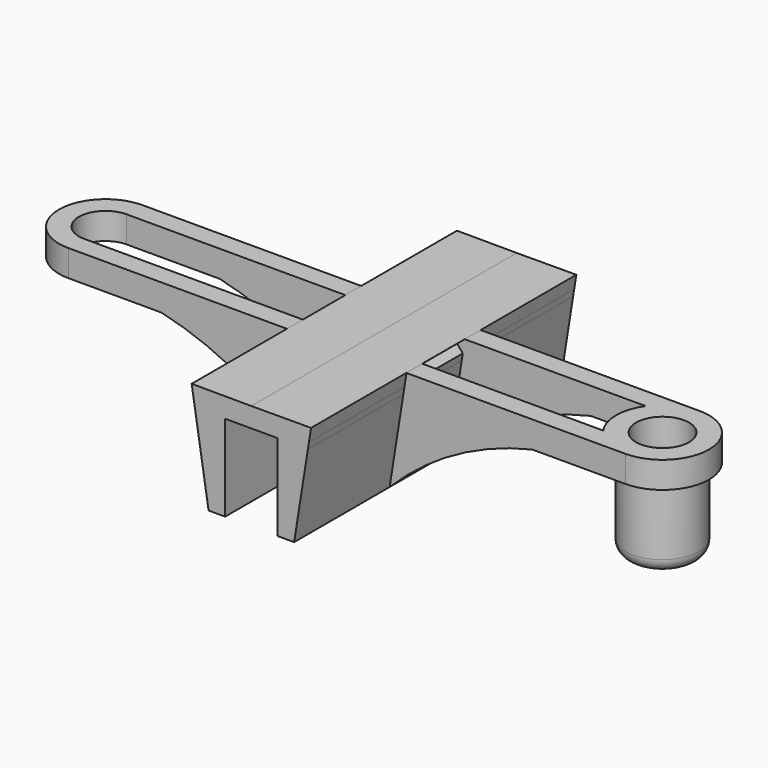
from build123d import *

# Parameters (mm, degrees)
F2_DEPTH  = 25
F3_DEPTH  = 4
F5_R      = 2
F6_DEPTH  = 18
F10_DEPTH = 3
F13_DEPTH = 3


# Not quite as in the source:
# - a feature names something its author has since deleted; it is built from what else it names


with BuildPart() as f2:
    # F0 (on Front) → F2 (new body, symmetric)
    with BuildSketch(Plane.XZ):
        Polygon((-3.95, -2.9709123753), (0, -2.9709123753), (0, 0), (-9, 0.0290876247), (-7.8289458158, -0.965005679), (-8.6815025112, -1.9693279914), (-8.521875, -2.9709123753), align=None)
        Polygon((3.95, -2.9709123753), (8.521875, -2.9709123753), (8.6815025112, -1.9693279914), (7.8289458158, -0.965005679), (9, 0.0290876247), (0, 0), (0, -2.9709123753), align=None)
        Polygon((-3.95, -15.9709123753), (-3.95, -2.9709123753), (-8.521875, -2.9709123753), (-6.45, -15.9709123753), align=None)
        Polygon((3.95, -15.9709123753), (6.45, -15.9709123753), (8.521875, -2.9709123753), (3.95, -2.9709123753), align=None)
    extrude(amount=F2_DEPTH, both=True)



with BuildPart() as f3:
    # F1 (on Top) → F3 (new body)
    with BuildSketch(Plane.XY):
        with BuildLine():
            ThreePointArc((42, -7), (49, 0), (42, 7))
            ThreePointArc((42, 7), (38.7596296508, 6.204836823), (36.2554373535, 4))
            Line((36.2554373535, 4), (42, 4))
            ThreePointArc((42, 4), (46, 0), (42, -4))
            Line((42, -4), (36.2554373535, -4))
            ThreePointArc((36.2554373535, -4), (38.7596296508, -6.204836823), (42, -7))
        make_face()
        with BuildLine():
            Line((7.5, -7), (9, -7))
            Line((9, -7), (42, -7))
            ThreePointArc((42, -7), (38.7596296508, -6.204836823), (36.2554373535, -4))
            Line((36.2554373535, -4), (9, -4))
            Line((9, -4), (7.5, -4))
            Line((7.5, -4), (7.5, -7))
        make_face()
        with BuildLine():
            Line((42, 7), (9, 7))
            Line((9, 7), (7.5, 7))
            Line((7.5, 7), (7.5, 4))
            Line((7.5, 4), (9, 4))
            Line((9, 4), (36.2554373535, 4))
            ThreePointArc((36.2554373535, 4), (38.7596296508, 6.204836823), (42, 7))
        make_face()
        with BuildLine():
            Line((42, 4), (36.2554373535, 4))
            ThreePointArc((36.2554373535, 4), (35, 0), (36.2554373535, -4))
            Line((36.2554373535, -4), (42, -4))
            ThreePointArc((42, -4), (38, 0), (42, 4))
        make_face()
    extrude(amount=-F3_DEPTH)


with BuildPart() as f3b:
    # F1 (on Top) → F3, piece 2 (new body)
    with BuildSketch(Plane.XY):
        with BuildLine():
            Line((-7.5, 7), (-9, 7))
            Line((-9, 7), (-42, 7))
            ThreePointArc((-42, 7), (-49, 0), (-42, -7))
            Line((-42, -7), (-9, -7))
            Line((-9, -7), (-7.5, -7))
            Line((-7.5, -7), (-7.5, -4))
            Line((-7.5, -4), (-9, -4))
            Line((-9, -4), (-42, -4))
            ThreePointArc((-42, -4), (-46, 0), (-42, 4))
            Line((-42, 4), (-9, 4))
            Line((-9, 4), (-7.5, 4))
            Line((-7.5, 4), (-7.5, 7))
        make_face()
    extrude(amount=-F3_DEPTH)


with BuildPart() as f2_1:
    add(f2.part)

    add(f3.part)  # F4 merges F3

    add(f3b.part)  # F4 merges F3b
    # F0 (on Front) → F4 (revolve)
    with BuildSketch(Plane.XZ):
        Polygon((47.506644696, -2.9709123753), (46, -2.9709123753), (45.9813326597, -14.9709123753), (43.4829847983, -14.9670259162), (43.4813326597, -16.0290766507), (47.506644696, -16.0290766507), align=None)
    revolve(axis=Axis((41.9813326597, 0, -8.0145383254), (0, 0, -1)))

    # F5
    f5_edges = [f2_1.edges().sort_by_distance(p)[0] for p in [
        (36.456021, 0, -16.029077),
    ]]
    fillet(f5_edges, radius=F5_R)



with BuildPart() as f6:
    # F0 (on Front) → F6 (new body)
    with BuildSketch(Plane.XZ):
        Polygon((7.8289458158, -0.965005679), (8.6815025112, -1.9693279914), (9, 0.0290876247), align=None)
    extrude(amount=F6_DEPTH)


with BuildPart() as f6_1:
    # F7: moved
    add(f6.part.moved(Location((0, -7, 0))))


with BuildPart() as f8_1:
    # F8: instance of F6
    add(f6_1.part.mirror(Plane.XZ))


with BuildPart() as f9_1:
    # F9: instance of F6
    add(f6_1.part.mirror(Plane.YZ))


with BuildPart() as f9_2:
    # F9: instance of F8_1
    add(f8_1.part.mirror(Plane.YZ))


with BuildPart() as f10:
    # F0 (on Front) → F10 (new body)
    with BuildSketch(Plane.XZ):
        with BuildLine():
            Line((8.521875, -2.9709123753), (6.45, -15.9709123753))
            ThreePointArc((6.45, -15.9709123753), (19.5335872752, -6.8543867374), (35, -2.9709123753))
            Line((35, -2.9709123753), (8.521875, -2.9709123753))
        make_face()
    extrude(amount=F10_DEPTH)


with BuildPart() as f10_1:
    # F11: moved
    add(f10.part.moved(Location((0, -4, 0))))


with BuildPart() as f2_2:
    add(f2_1.part)

    add(f6_1.part)  # F12 merges F6

    add(f8_1.part)  # F12 merges F8_1

    add(f9_1.part)  # F12 merges F9_1

    add(f9_2.part)  # F12 merges F9_2

    add(f10_1.part)  # F12 merges F10
    # F12: F10 across plane
    add(f10_1.part.mirror(Plane.XZ))



with BuildPart() as f13:
    # F0 (on Front) → F13 (new body)
    with BuildSketch(Plane.XZ):
        with BuildLine():
            Line((-6.45, -15.9709123753), (-8.521875, -2.9709123753))
            Line((-8.521875, -2.9709123753), (-35, -2.9709123753))
            ThreePointArc((-35, -2.9709123753), (-19.5335872752, -6.8543867374), (-6.45, -15.9709123753))
        make_face()
    extrude(amount=F13_DEPTH)


with BuildPart() as f13_1:
    # F14: moved
    add(f13.part.moved(Location((0, -4, 0))))


with BuildPart() as f2_3:
    add(f2_2.part)

    add(f13_1.part)  # F15 merges F13
    # F15: F13 across plane
    add(f13_1.part.mirror(Plane.XZ))


solid = f2_3.part
